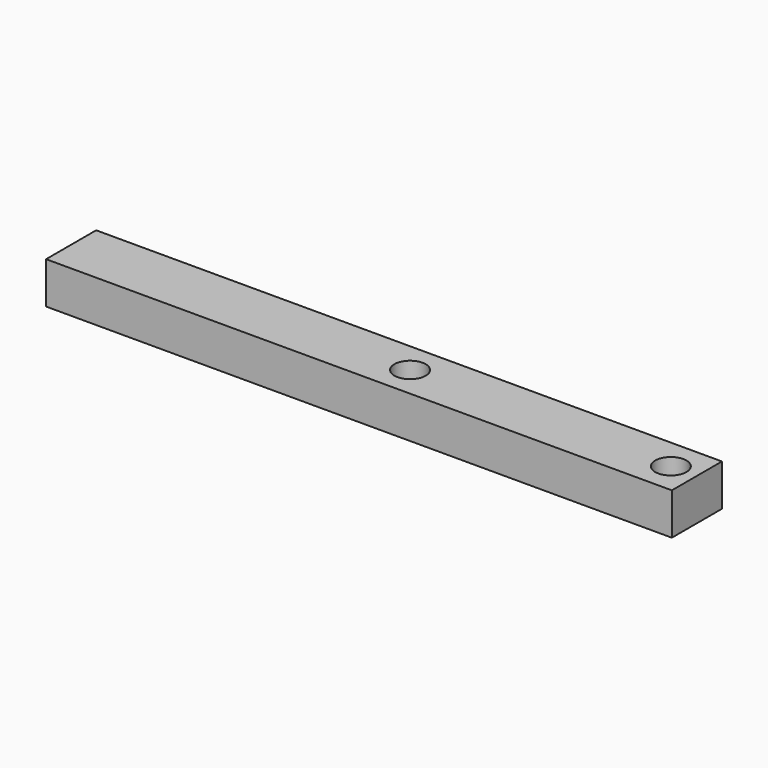
from build123d import *

# Parameters (mm, degrees)
F1_DEPTH = 4
F2_D     = 3


# Not quite as in the source:
# - a feature names something its author has since deleted; it is built from what else it names


with BuildPart() as f1:
    # F0 (on Top) → F1 (new body)
    with BuildSketch(Plane.XY):
        Polygon((-17.5, -3), (42.5, -3), (42.5, 0), (42.5, 3), (-17.5, 3), (-17.5, 0), align=None)
    extrude(amount=F1_DEPTH)

    # F2 (through all)
    with Locations(Plane(origin=(0, 0, 0), x_dir=(1, 0, 0), z_dir=(0, 0, -1))):
        with Locations((40, 0), (15, 0)):
            Hole(F2_D / 2)


solid = f1.part
